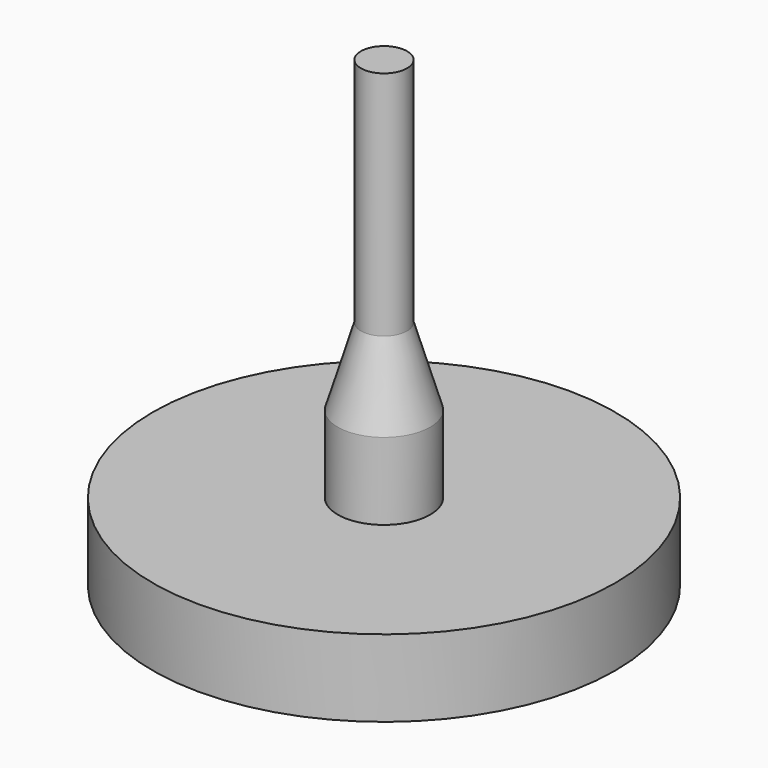
from build123d import *

# Parameters (mm, degrees)
F0_R     = 38.1
F1_DEPTH = 12.7
F2_R     = 7.62
F3_DEPTH = 12.7
F6_DEPTH = 38.1


# Not quite as in the source:
# - a feature names something its author has since deleted; it is built from what else it names


with BuildPart() as f1:
    # F0 (on Top) → F1 (new body)
    with BuildSketch(Plane.XY):
        Circle(F0_R)
    extrude(amount=F1_DEPTH)

    # F2 (on face) → F3 (join)
    with BuildSketch(Plane.XY.offset(12.7)):
        Circle(F2_R)
    extrude(amount=F3_DEPTH)

    # F4 (on Right) → F5 (revolve)
    with BuildSketch(Plane.YZ):
        Polygon((0, 38.1), (0, 25.4), (7.62, 25.4), (3.81, 38.1), align=None)
    revolve(axis=Axis((0, 0, 31.75), (0, 0, 1)))

    # F6 (add): a face of the model
    f6_faces = [f1.faces().sort_by_distance(p)[0] for p in [
        (0, 0, 38.1),
    ]]
    extrude(f6_faces, amount=F6_DEPTH)


solid = f1.part
